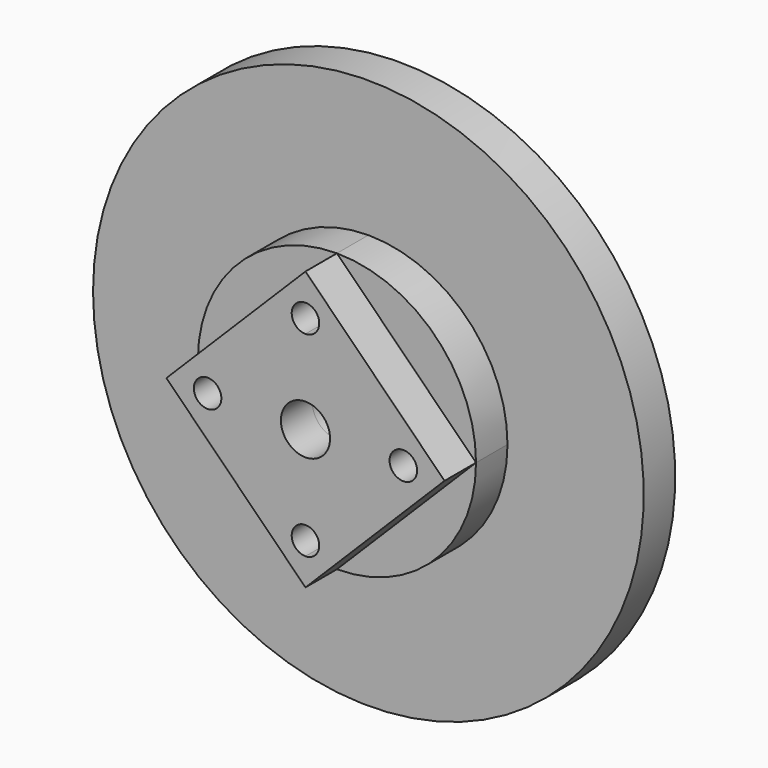
from build123d import *
from build123d import SkipClean  # not in build123d's __all__

# Parameters (mm, degrees)
F0_R      = 35.18
F0_R_2    = 12.5
F1_DEPTH  = 20
F2_DEPTH  = 15
F3_DEPTH  = 20
F0_R_3    = 9.5
F6_DEPTH  = 92
F7_R      = 9.5
F8_DEPTH  = 70
F9_W      = 11.313708499
F9_H      = 11.313708499
F10_DEPTH = 20
F9_R      = 10
F11_DEPTH = 10


# Not quite as in the source:
# - after a boolean that leaves OpenCascade's solid faulty, fix() repairs it


with BuildPart() as f1:
    # F0 (on Front) → F1 (new body)
    with BuildSketch(Plane.XZ):
        with BuildLine():
            Line((63.298904413, -7.4117737057), (70.7106781187, 0))
            Line((70.7106781187, 0), (63.298904413, 7.4117737057))
            ThreePointArc((63.298904413, 7.4117737057), (63.6231509631, 3.7121894992), (63.7313556215, 0))
            ThreePointArc((63.7313556215, 0), (63.6231509631, -3.7121894992), (63.298904413, -7.4117737057))
        make_face()
        with BuildLine():
            ThreePointArc((63.7313556215, 0), (63.6231509631, 3.7121894992), (63.298904413, 7.4117737057))
            Line((63.298904413, 7.4117737057), (54.3394543105, 16.3712238082))
            ThreePointArc((54.3394543105, 16.3712238082), (56.1456488729, 8.2740181519), (56.7520331243, 0))
            ThreePointArc((56.7520331243, 0), (56.1456488729, -8.2740181519), (54.3394543105, -16.3712238082))
            Line((54.3394543105, -16.3712238082), (63.298904413, -7.4117737057))
            ThreePointArc((63.298904413, -7.4117737057), (63.6231509631, -3.7121894992), (63.7313556215, 0))
        make_face()
        with BuildLine():
            ThreePointArc((56.7520331243, 0), (56.1456488729, 8.2740181519), (54.3394543105, 16.3712238082))
            Line((54.3394543105, 16.3712238082), (16.3712238082, 54.3394543105))
            ThreePointArc((16.3712238082, 54.3394543105), (8.274018171, 56.1456488701), (3.86e-08, 56.7520331243))
            ThreePointArc((3.86e-08, 56.7520331243), (4.949747482, 54.7017805789), (7, 49.7520331243))
            ThreePointArc((7, 49.7520331243), (4.9497474448, 44.8022856325), (-6.65e-08, 42.7520331243))
            ThreePointArc((-6.65e-08, 42.7520331243), (30.2302525082, 30.2302525552), (42.7520331243, 0))
            ThreePointArc((42.7520331243, 0), (49.7520331243, 7), (56.7520331243, 0))
        make_face()
        with BuildLine():
            Line((16.3712238082, 54.3394543105), (7.4117737057, 63.298904413))
            ThreePointArc((7.4117737057, 63.298904413), (0, 63.7313556215), (-7.4117737057, 63.298904413))
            Line((-7.4117737057, 63.298904413), (-16.3712238082, 54.3394543105))
            ThreePointArc((-16.3712238082, 54.3394543105), (-8.2740181328, 56.1456488757), (3.86e-08, 56.7520331243))
            ThreePointArc((3.86e-08, 56.7520331243), (8.274018171, 56.1456488701), (16.3712238082, 54.3394543105))
        make_face()
        with BuildLine():
            Line((7.4117737057, 63.298904413), (0, 70.7106781187))
            Line((0, 70.7106781187), (-7.4117737057, 63.298904413))
            ThreePointArc((-7.4117737057, 63.298904413), (0, 63.7313556215), (7.4117737057, 63.298904413))
        make_face()
        with BuildLine():
            ThreePointArc((3.86e-08, 56.7520331243), (-8.2740181328, 56.1456488757), (-16.3712238082, 54.3394543105))
            Line((-16.3712238082, 54.3394543105), (-54.3394543105, 16.3712238082))
            ThreePointArc((-54.3394543105, 16.3712238082), (-56.1456488729, 8.2740181519), (-56.7520331243, 0))
            ThreePointArc((-56.7520331243, 0), (-49.7520331243, 7), (-42.7520331243, 0))
            ThreePointArc((-42.7520331243, 0), (-30.2302525552, 30.2302525082), (-6.65e-08, 42.7520331243))
            ThreePointArc((-6.65e-08, 42.7520331243), (-7, 49.7520331768), (3.86e-08, 56.7520331243))
        make_face()
        with BuildLine():
            ThreePointArc((3.55e-08, -42.7520331243), (30.2302525443, -30.2302525191), (42.7520331243, 0))
            ThreePointArc((42.7520331243, 0), (30.2302525082, 30.2302525552), (-6.65e-08, 42.7520331243))
            ThreePointArc((-6.65e-08, 42.7520331243), (-30.2302525552, 30.2302525082), (-42.7520331243, 0))
            ThreePointArc((-42.7520331243, 0), (-30.2302525191, -30.2302525443), (3.55e-08, -42.7520331243))
        make_face()
        Circle(F0_R, mode=Mode.SUBTRACT)
        with BuildLine():
            Line((16.3712238082, -54.3394543105), (54.3394543105, -16.3712238082))
            ThreePointArc((54.3394543105, -16.3712238082), (56.1456488729, -8.2740181519), (56.7520331243, 0))
            ThreePointArc((56.7520331243, 0), (49.7520331243, -7), (42.7520331243, 0))
            ThreePointArc((42.7520331243, 0), (30.2302525443, -30.2302525191), (3.55e-08, -42.7520331243))
            ThreePointArc((3.55e-08, -42.7520331243), (4.9497474809, -44.8022856685), (7, -49.7520331243))
            ThreePointArc((7, -49.7520331243), (4.9497475177, -54.7017805432), (1.398e-07, -56.7520331243))
            ThreePointArc((1.398e-07, -56.7520331243), (8.274018221, -56.1456488627), (16.3712238082, -54.3394543105))
        make_face()
        with BuildLine():
            Line((-54.3394543105, -16.3712238082), (-16.3712238082, -54.3394543105))
            ThreePointArc((-16.3712238082, -54.3394543105), (-8.2740180827, -56.1456488831), (1.398e-07, -56.7520331243))
            ThreePointArc((1.398e-07, -56.7520331243), (-7, -49.7520331764), (3.55e-08, -42.7520331243))
            ThreePointArc((3.55e-08, -42.7520331243), (-30.2302525191, -30.2302525443), (-42.7520331243, 0))
            ThreePointArc((-42.7520331243, 0), (-49.7520331243, -7), (-56.7520331243, 0))
            ThreePointArc((-56.7520331243, 0), (-56.1456488729, -8.2740181519), (-54.3394543105, -16.3712238082))
        make_face()
        with BuildLine():
            ThreePointArc((-7.4117737057, -63.298904413), (0, -63.7313556215), (7.4117737057, -63.298904413))
            Line((7.4117737057, -63.298904413), (16.3712238082, -54.3394543105))
            ThreePointArc((16.3712238082, -54.3394543105), (8.274018221, -56.1456488627), (1.398e-07, -56.7520331243))
            ThreePointArc((1.398e-07, -56.7520331243), (-8.2740180827, -56.1456488831), (-16.3712238082, -54.3394543105))
            Line((-16.3712238082, -54.3394543105), (-7.4117737057, -63.298904413))
        make_face()
        with BuildLine():
            Line((-7.4117737057, -63.298904413), (0, -70.7106781187))
            Line((0, -70.7106781187), (7.4117737057, -63.298904413))
            ThreePointArc((7.4117737057, -63.298904413), (0, -63.7313556215), (-7.4117737057, -63.298904413))
        make_face()
        with BuildLine():
            Line((-54.3394543105, 16.3712238082), (-63.298904413, 7.4117737057))
            ThreePointArc((-63.298904413, 7.4117737057), (-63.7313556215, 0), (-63.298904413, -7.4117737057))
            Line((-63.298904413, -7.4117737057), (-54.3394543105, -16.3712238082))
            ThreePointArc((-54.3394543105, -16.3712238082), (-56.1456488729, -8.2740181519), (-56.7520331243, 0))
            ThreePointArc((-56.7520331243, 0), (-56.1456488729, 8.2740181519), (-54.3394543105, 16.3712238082))
        make_face()
        with BuildLine():
            Line((-63.298904413, 7.4117737057), (-70.7106781187, 0))
            Line((-70.7106781187, 0), (-63.298904413, -7.4117737057))
            ThreePointArc((-63.298904413, -7.4117737057), (-63.7313556215, 0), (-63.298904413, 7.4117737057))
        make_face()
        Circle(F0_R)
        Circle(F0_R_2, mode=Mode.SUBTRACT)
    extrude(amount=F1_DEPTH)

    # F0 (on Front) → F2 (join)
    with BuildSketch(Plane.XZ):
        Circle(F0_R)
        Circle(F0_R_2, mode=Mode.SUBTRACT)
    extrude(amount=-F2_DEPTH)

    # F0 (on Front) → F3 (join)
    with BuildSketch(Plane.XZ):
        with BuildLine():
            ThreePointArc((3.55e-08, -42.7520331243), (30.2302525443, -30.2302525191), (42.7520331243, 0))
            ThreePointArc((42.7520331243, 0), (30.2302525082, 30.2302525552), (-6.65e-08, 42.7520331243))
            ThreePointArc((-6.65e-08, 42.7520331243), (-30.2302525552, 30.2302525082), (-42.7520331243, 0))
            ThreePointArc((-42.7520331243, 0), (-30.2302525191, -30.2302525443), (3.55e-08, -42.7520331243))
        make_face()
        Circle(F0_R, mode=Mode.SUBTRACT)
        with BuildLine():
            Line((16.3712238082, -54.3394543105), (54.3394543105, -16.3712238082))
            ThreePointArc((54.3394543105, -16.3712238082), (56.1456488729, -8.2740181519), (56.7520331243, 0))
            ThreePointArc((56.7520331243, 0), (49.7520331243, -7), (42.7520331243, 0))
            ThreePointArc((42.7520331243, 0), (30.2302525443, -30.2302525191), (3.55e-08, -42.7520331243))
            ThreePointArc((3.55e-08, -42.7520331243), (4.9497474809, -44.8022856685), (7, -49.7520331243))
            ThreePointArc((7, -49.7520331243), (4.9497475177, -54.7017805432), (1.398e-07, -56.7520331243))
            ThreePointArc((1.398e-07, -56.7520331243), (8.274018221, -56.1456488627), (16.3712238082, -54.3394543105))
        make_face()
        with BuildLine():
            ThreePointArc((16.3712238082, -54.3394543105), (40.1297474683, -40.1297474683), (54.3394543105, -16.3712238082))
            Line((54.3394543105, -16.3712238082), (16.3712238082, -54.3394543105))
        make_face()
        with BuildLine():
            ThreePointArc((7.4117737057, -63.298904413), (45.0648737342, -45.0648737342), (63.298904413, -7.4117737057))
            Line((63.298904413, -7.4117737057), (54.3394543105, -16.3712238082))
            ThreePointArc((54.3394543105, -16.3712238082), (40.1297474683, -40.1297474683), (16.3712238082, -54.3394543105))
            Line((16.3712238082, -54.3394543105), (7.4117737057, -63.298904413))
        make_face()
        with BuildLine():
            ThreePointArc((0, -70.7106781187), (50, -50), (70.7106781187, 0))
            Line((70.7106781187, 0), (63.298904413, -7.4117737057))
            ThreePointArc((63.298904413, -7.4117737057), (45.0648737342, -45.0648737342), (7.4117737057, -63.298904413))
            Line((7.4117737057, -63.298904413), (0, -70.7106781187))
        make_face()
        with BuildLine():
            ThreePointArc((63.7313556215, 0), (63.6231509631, 3.7121894992), (63.298904413, 7.4117737057))
            Line((63.298904413, 7.4117737057), (54.3394543105, 16.3712238082))
            ThreePointArc((54.3394543105, 16.3712238082), (56.1456488729, 8.2740181519), (56.7520331243, 0))
            ThreePointArc((56.7520331243, 0), (56.1456488729, -8.2740181519), (54.3394543105, -16.3712238082))
            Line((54.3394543105, -16.3712238082), (63.298904413, -7.4117737057))
            ThreePointArc((63.298904413, -7.4117737057), (63.6231509631, -3.7121894992), (63.7313556215, 0))
        make_face()
        with BuildLine():
            Line((63.298904413, -7.4117737057), (70.7106781187, 0))
            Line((70.7106781187, 0), (63.298904413, 7.4117737057))
            ThreePointArc((63.298904413, 7.4117737057), (63.6231509631, 3.7121894992), (63.7313556215, 0))
            ThreePointArc((63.7313556215, 0), (63.6231509631, -3.7121894992), (63.298904413, -7.4117737057))
        make_face()
        with BuildLine():
            Line((63.298904413, 7.4117737057), (70.7106781187, 0))
            ThreePointArc((70.7106781187, 0), (50, 50), (0, 70.7106781187))
            Line((0, 70.7106781187), (7.4117737057, 63.298904413))
            ThreePointArc((7.4117737057, 63.298904413), (45.0648737342, 45.0648737342), (63.298904413, 7.4117737057))
        make_face()
        with BuildLine():
            Line((54.3394543105, 16.3712238082), (63.298904413, 7.4117737057))
            ThreePointArc((63.298904413, 7.4117737057), (45.0648737342, 45.0648737342), (7.4117737057, 63.298904413))
            Line((7.4117737057, 63.298904413), (16.3712238082, 54.3394543105))
            ThreePointArc((16.3712238082, 54.3394543105), (40.1297474683, 40.1297474683), (54.3394543105, 16.3712238082))
        make_face()
        with BuildLine():
            Line((16.3712238082, 54.3394543105), (54.3394543105, 16.3712238082))
            ThreePointArc((54.3394543105, 16.3712238082), (40.1297474683, 40.1297474683), (16.3712238082, 54.3394543105))
        make_face()
        with BuildLine():
            ThreePointArc((56.7520331243, 0), (56.1456488729, 8.2740181519), (54.3394543105, 16.3712238082))
            Line((54.3394543105, 16.3712238082), (16.3712238082, 54.3394543105))
            ThreePointArc((16.3712238082, 54.3394543105), (8.274018171, 56.1456488701), (3.86e-08, 56.7520331243))
            ThreePointArc((3.86e-08, 56.7520331243), (4.949747482, 54.7017805789), (7, 49.7520331243))
            ThreePointArc((7, 49.7520331243), (4.9497474448, 44.8022856325), (-6.65e-08, 42.7520331243))
            ThreePointArc((-6.65e-08, 42.7520331243), (30.2302525082, 30.2302525552), (42.7520331243, 0))
            ThreePointArc((42.7520331243, 0), (49.7520331243, 7), (56.7520331243, 0))
        make_face()
        with BuildLine():
            Line((16.3712238082, 54.3394543105), (7.4117737057, 63.298904413))
            ThreePointArc((7.4117737057, 63.298904413), (0, 63.7313556215), (-7.4117737057, 63.298904413))
            Line((-7.4117737057, 63.298904413), (-16.3712238082, 54.3394543105))
            ThreePointArc((-16.3712238082, 54.3394543105), (-8.2740181328, 56.1456488757), (3.86e-08, 56.7520331243))
            ThreePointArc((3.86e-08, 56.7520331243), (8.274018171, 56.1456488701), (16.3712238082, 54.3394543105))
        make_face()
        with BuildLine():
            Line((7.4117737057, 63.298904413), (0, 70.7106781187))
            Line((0, 70.7106781187), (-7.4117737057, 63.298904413))
            ThreePointArc((-7.4117737057, 63.298904413), (0, 63.7313556215), (7.4117737057, 63.298904413))
        make_face()
        with BuildLine():
            Line((-16.3712238082, 54.3394543105), (-7.4117737057, 63.298904413))
            ThreePointArc((-7.4117737057, 63.298904413), (-45.0648737342, 45.0648737342), (-63.298904413, 7.4117737057))
            Line((-63.298904413, 7.4117737057), (-54.3394543105, 16.3712238082))
            ThreePointArc((-54.3394543105, 16.3712238082), (-40.1297474683, 40.1297474683), (-16.3712238082, 54.3394543105))
        make_face()
        with BuildLine():
            Line((-54.3394543105, 16.3712238082), (-16.3712238082, 54.3394543105))
            ThreePointArc((-16.3712238082, 54.3394543105), (-40.1297474683, 40.1297474683), (-54.3394543105, 16.3712238082))
        make_face()
        with BuildLine():
            ThreePointArc((3.86e-08, 56.7520331243), (-8.2740181328, 56.1456488757), (-16.3712238082, 54.3394543105))
            Line((-16.3712238082, 54.3394543105), (-54.3394543105, 16.3712238082))
            ThreePointArc((-54.3394543105, 16.3712238082), (-56.1456488729, 8.2740181519), (-56.7520331243, 0))
            ThreePointArc((-56.7520331243, 0), (-49.7520331243, 7), (-42.7520331243, 0))
            ThreePointArc((-42.7520331243, 0), (-30.2302525552, 30.2302525082), (-6.65e-08, 42.7520331243))
            ThreePointArc((-6.65e-08, 42.7520331243), (-7, 49.7520331768), (3.86e-08, 56.7520331243))
        make_face()
        with BuildLine():
            Line((-7.4117737057, 63.298904413), (0, 70.7106781187))
            ThreePointArc((0, 70.7106781187), (-50, 50), (-70.7106781187, 0))
            Line((-70.7106781187, 0), (-63.298904413, 7.4117737057))
            ThreePointArc((-63.298904413, 7.4117737057), (-45.0648737342, 45.0648737342), (-7.4117737057, 63.298904413))
        make_face()
        with BuildLine():
            Line((-54.3394543105, 16.3712238082), (-63.298904413, 7.4117737057))
            ThreePointArc((-63.298904413, 7.4117737057), (-63.7313556215, 0), (-63.298904413, -7.4117737057))
            Line((-63.298904413, -7.4117737057), (-54.3394543105, -16.3712238082))
            ThreePointArc((-54.3394543105, -16.3712238082), (-56.1456488729, -8.2740181519), (-56.7520331243, 0))
            ThreePointArc((-56.7520331243, 0), (-56.1456488729, 8.2740181519), (-54.3394543105, 16.3712238082))
        make_face()
        with BuildLine():
            Line((-63.298904413, 7.4117737057), (-70.7106781187, 0))
            Line((-70.7106781187, 0), (-63.298904413, -7.4117737057))
            ThreePointArc((-63.298904413, -7.4117737057), (-63.7313556215, 0), (-63.298904413, 7.4117737057))
        make_face()
        with BuildLine():
            ThreePointArc((-70.7106781187, 0), (-50, -50), (0, -70.7106781187))
            Line((0, -70.7106781187), (-7.4117737057, -63.298904413))
            ThreePointArc((-7.4117737057, -63.298904413), (-45.0648737342, -45.0648737342), (-63.298904413, -7.4117737057))
            Line((-63.298904413, -7.4117737057), (-70.7106781187, 0))
        make_face()
        with BuildLine():
            ThreePointArc((-63.298904413, -7.4117737057), (-45.0648737342, -45.0648737342), (-7.4117737057, -63.298904413))
            Line((-7.4117737057, -63.298904413), (-16.3712238082, -54.3394543105))
            ThreePointArc((-16.3712238082, -54.3394543105), (-40.1297474683, -40.1297474683), (-54.3394543105, -16.3712238082))
            Line((-54.3394543105, -16.3712238082), (-63.298904413, -7.4117737057))
        make_face()
        with BuildLine():
            ThreePointArc((-54.3394543105, -16.3712238082), (-40.1297474683, -40.1297474683), (-16.3712238082, -54.3394543105))
            Line((-16.3712238082, -54.3394543105), (-54.3394543105, -16.3712238082))
        make_face()
        with BuildLine():
            Line((-54.3394543105, -16.3712238082), (-16.3712238082, -54.3394543105))
            ThreePointArc((-16.3712238082, -54.3394543105), (-8.2740180827, -56.1456488831), (1.398e-07, -56.7520331243))
            ThreePointArc((1.398e-07, -56.7520331243), (-7, -49.7520331764), (3.55e-08, -42.7520331243))
            ThreePointArc((3.55e-08, -42.7520331243), (-30.2302525191, -30.2302525443), (-42.7520331243, 0))
            ThreePointArc((-42.7520331243, 0), (-49.7520331243, -7), (-56.7520331243, 0))
            ThreePointArc((-56.7520331243, 0), (-56.1456488729, -8.2740181519), (-54.3394543105, -16.3712238082))
        make_face()
        with BuildLine():
            ThreePointArc((-7.4117737057, -63.298904413), (0, -63.7313556215), (7.4117737057, -63.298904413))
            Line((7.4117737057, -63.298904413), (16.3712238082, -54.3394543105))
            ThreePointArc((16.3712238082, -54.3394543105), (8.274018221, -56.1456488627), (1.398e-07, -56.7520331243))
            ThreePointArc((1.398e-07, -56.7520331243), (-8.2740180827, -56.1456488831), (-16.3712238082, -54.3394543105))
            Line((-16.3712238082, -54.3394543105), (-7.4117737057, -63.298904413))
        make_face()
        with BuildLine():
            Line((-7.4117737057, -63.298904413), (0, -70.7106781187))
            Line((0, -70.7106781187), (7.4117737057, -63.298904413))
            ThreePointArc((7.4117737057, -63.298904413), (0, -63.7313556215), (-7.4117737057, -63.298904413))
        make_face()
    with SkipClean():  # cleaning this boolean's faces spoils the solid; the shape is the same uncleaned
        extrude(amount=-F3_DEPTH)

    # F4 (on Top) → F5 (revolve)
    with BuildSketch(Plane.XY):
        Polygon((-84, 20), (-70.7106781187, 20), (-63.7313556215, 20), (-63.7313556215, 40), (-140, 40), (-140, 20), (-103, 20), align=None)
    revolve(axis=Axis((0, 0, 0), (0, 1, 0)))

    add(f1.part.fix(), mode=Mode.REPLACE)

    # F0 (on Front) → F6 (cut)
    with BuildSketch(Plane.XZ):
        with Locations((-93.5, 0)):
            Circle(F0_R_3)
    extrude(amount=-F6_DEPTH, mode=Mode.SUBTRACT)

    # F7 (on face) → F8 (join)
    with BuildSketch(Plane.XZ.offset(-20)):
        with Locations((-93.5, 0)):
            Circle(F7_R)
    extrude(amount=-F8_DEPTH)

    # F9 (on face) → F10 (join)
    with BuildSketch(Plane(origin=(0, 90, 0), x_dir=(-1, 0, 0), z_dir=(0, 1, 0))):
        with Locations((93.5, 0)):
            Rectangle(F9_W, F9_H)
    extrude(amount=F10_DEPTH)

    # F9 (on face) → F11 (join)
    with BuildSketch(Plane(origin=(0, 90, 0), x_dir=(-1, 0, 0), z_dir=(0, 1, 0))):
        with Locations((93.5, 0)):
            Circle(F9_R)
        with Locations((93.5, 0)):
            Rectangle(F9_W, F9_H, mode=Mode.SUBTRACT)
    extrude(amount=F11_DEPTH)


solid = f1.part
